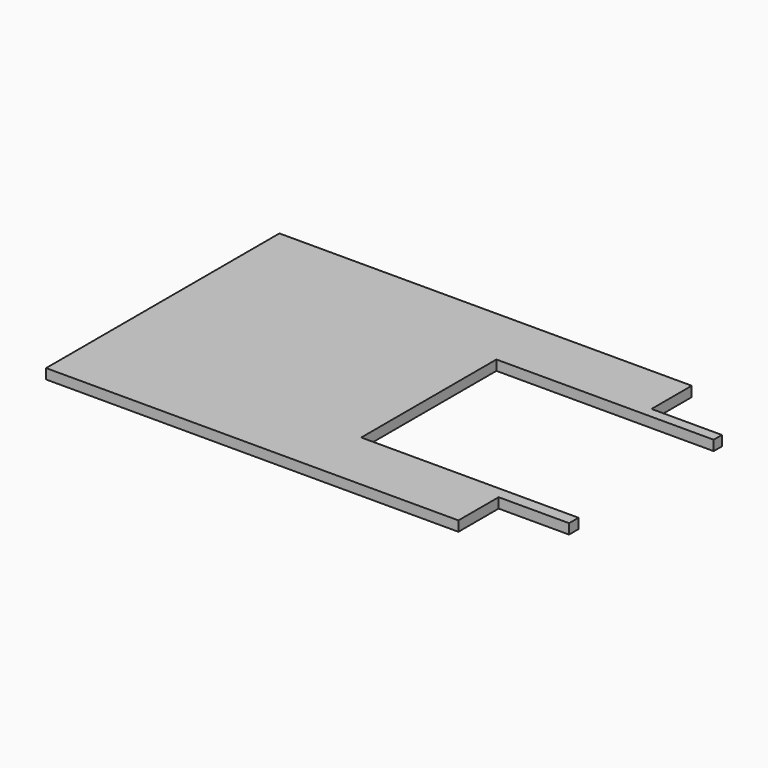
from build123d import *

# Parameters (mm, degrees)
F1_DEPTH = 3.175


# Not quite as in the source:
# - a length typed as a fraction of an inch, garbled in the dataset ("3 / 203.2 mm" for 3/8 in), is restored


with BuildPart() as f1:
    # F0 (on Top) → F1 (new body)
    with BuildSketch(Plane.XY):
        Polygon((-42.3513493031, 87.8042607932), (-172.5263493031, 87.8042607932), (-172.5263493031, -4.2707392068), (-42.3513493031, -4.2707392068), (-42.3513493031, 11.6042607932), (-20.1263493031, 11.6042607932), (-20.1263493031, 15.3254829347), (-88.7063493031, 15.3254829347), (-88.7063493031, 68.6654829347), (-20.1263493031, 68.6654829347), (-20.1263493031, 71.9292607932), (-42.3513493031, 71.9292607932), align=None)
    extrude(amount=-F1_DEPTH)


solid = f1.part
